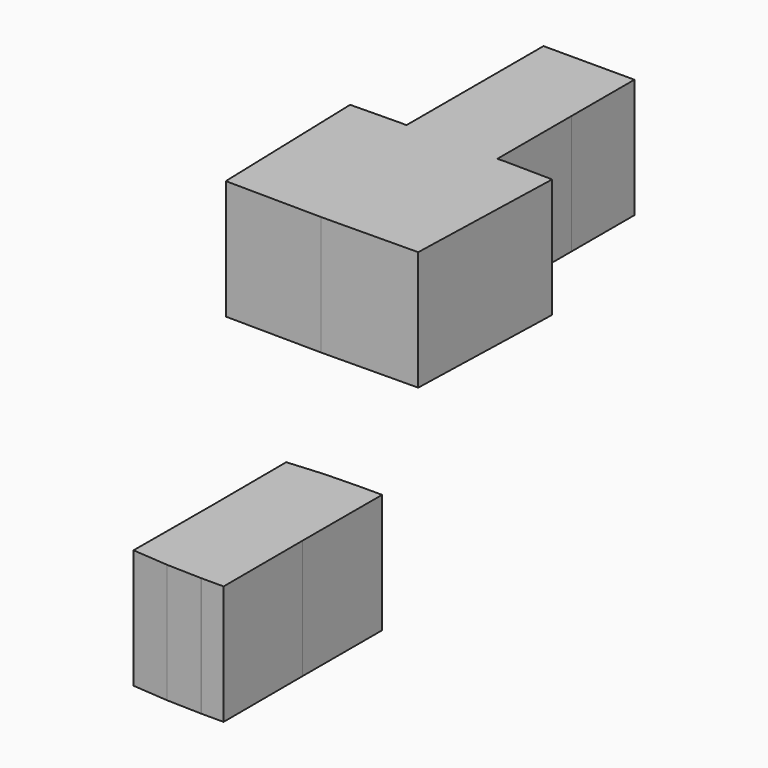
from build123d import *

# Parameters (mm, degrees)
F1_DEPTH = 12.7
F2_DEPTH = 12.7
F3_DEPTH = 12.7


# Not quite as in the source:
# - ends of sketch curves that miss each other by under 0.0002 mm in the source are joined


with BuildPart() as f1:
    # F0 (on Top) → F1 (new body)
    with BuildSketch(Plane.XY):
        Polygon((48.1904364, -56.783518093), (44.3699114476, -57.0827370893), (44.4090344471, -67.2408419628), (44.3699114476, -77.3989428363), (48.1680944003, -77.6981328326), (51.8766943541, -77.8051478313), (51.9053793534, -77.8051322055), (54.2796933242, -77.8038388313), (54.2560783245, -67.2473299627), (54.2674333243, -56.6907980942), (51.8931293539, -56.6922220942), align=None)
    extrude(amount=F1_DEPTH)


with BuildPart() as f2:
    # F0 (on Top) → F2 (new body)
    with BuildSketch(Plane.XY):
        Polygon((19.0754927625, -3.3519267583), (14.2665940583, -3.4246807871), (14.2665828224, -3.4606557569), (13.6578667858, -3.4338902474), (8.3214078964, -3.5146257562), (8.83126389, -20.7016265423), (19.0754967625, -20.8079195409), (29.319728635, -20.7016265423), (29.8295716286, -3.5146237562), (24.5883054068, -3.4353293517), (23.9535827018, -3.4629397569), (23.9535885865, -3.4257268072), align=None)
    extrude(amount=F2_DEPTH)

    # F0 (on Top) → F3 (join)
    with BuildSketch(Plane.XY):
        Polygon((14.2716398223, 14.781595016), (14.2696678223, 6.4168211201), (14.2665940583, -3.4246807871), (19.0754927625, -3.3519267583), (23.9535885865, -3.4257268072), (23.9551447017, 6.4145411201), (23.9571087017, 14.779316016), (19.114378762, 14.780459016), align=None)
    extrude(amount=F3_DEPTH)


solid = Compound([f1.part, f2.part])
